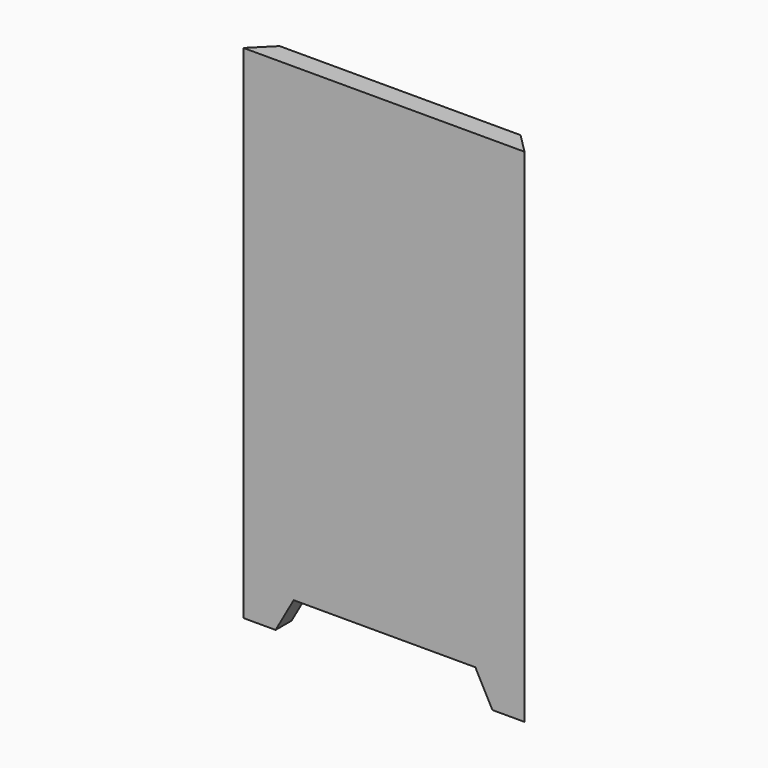
from build123d import *

# Parameters (mm, degrees)
F1_DEPTH = 10
F2_SIZE  = 9.99999


# Not quite as in the source:
# - a fillet or chamfer is up to 0.001 mm smaller than in the source, because OpenCascade refuses the exact size


with BuildPart() as f1:
    # F0 (on Front) → F1 (new body)
    with BuildSketch(Plane.XZ):
        Polygon((70, -108.8627894558), (70, 125), (-70, 125), (-70, -125), (-54, -125), (-45, -109.0002581477), (45.5037690699, -109.0002581477), (54, -125), (70, -125), align=None)
    extrude(amount=F1_DEPTH)

    # F2 (size 10 in the source; OpenCascade refuses exactly that, so slightly less here)
    f2_edges = [f1.edges().sort_by_distance(p)[0] for p in [
        (-70, 0, 0),
        (70, 0, 0),
    ]]
    chamfer(f2_edges, length=F2_SIZE)


solid = f1.part
